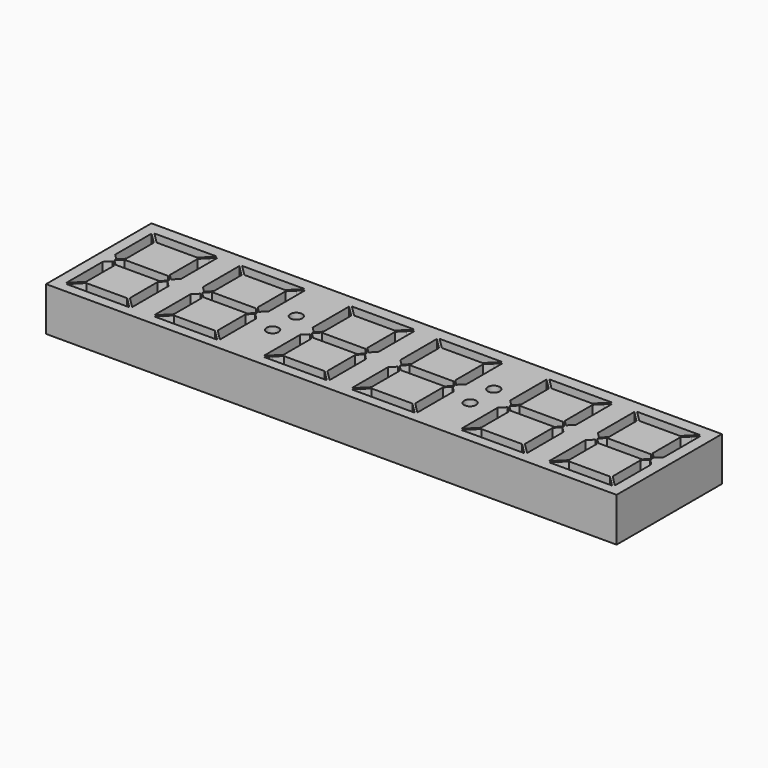
from build123d import *

# Parameters (mm, degrees)
F0_R     = 3.4648968079
F1_DEPTH = 25.4


# Not quite as in the source:
# - ends of sketch curves that miss each other by under 0.0002 mm in the source are joined


with BuildPart() as f1:
    # F0 (on Top) → F1 (new body)
    with BuildSketch(Plane.XY):
        Polygon((-45.9224169783, 52.1854245931), (-71.324658747, 52.1854245931), (-122.124658747, 52.1854245931), (-122.124658747, -24.0145754069), (-71.324658747, -24.0145754069), (-20.5201752096, -24.0145754069), (-7.824658747, -24.0145754069), (-7.8201752096, -24.0145754069), (42.975341253, -24.0145754069), (93.7798247904, -24.0145754069), (106.475341253, -24.0145754069), (106.4798247904, -24.0145754069), (157.275341253, -24.0145754069), (208.0798247904, -24.0145754069), (208.0798247904, 52.1854245931), (182.6775830217, 52.1854245931), (157.275341253, 52.1854245931), (106.4798247904, 52.1854245931), (106.475341253, 52.1854245931), (100.1298247904, 52.1854245931), (93.7798247904, 52.1854245931), (68.3775830217, 52.1854245931), (42.975341253, 52.1854245931), (-7.8201752096, 52.1854245931), (-7.824658747, 52.1854245931), (-14.1701752096, 52.1854245931), (-20.5201752096, 52.1854245931), align=None)
        Polygon((-114.8766638426, -18.2225372752), (-112.1506766486, -15.4965500813), (-108.5266638426, -11.8725372752), (-84.9227150668, -11.8725372752), (-81.2987022607, -15.4965500813), (-78.5727150668, -18.2225372752), align=None, mode=Mode.SUBTRACT)
        Polygon((-27.7726536514, -18.2225372752), (-64.0766024272, -18.2225372752), (-61.3506152332, -15.4965500813), (-57.7266024272, -11.8725372752), (-34.1226536514, -11.8725372752), (-30.4986408454, -15.4965500813), align=None, mode=Mode.SUBTRACT)
        Polygon((5.7733361574, -11.8725372752), (29.3772849332, -11.8725372752), (33.0012977393, -15.4965500813), (35.7272849332, -18.2225372752), (-0.5766638426, -18.2225372752), (2.1493233514, -15.4965500813), align=None, mode=Mode.SUBTRACT)
        Polygon((-115.7770073018, 9.0053659809), (-115.7061190955, 9.0824627244), (-112.5653735672, 12.2574627244), (-109.4246280391, 9.0824627243), (-109.4246280391, -10.9745116633), (-113.0486408451, -14.5985244694), (-115.7746284012, -17.3245116571), align=None, mode=Mode.SUBTRACT)
        Polygon((-80.8810682654, 12.2546509709), (-77.7403227372, 9.0796509709), (-77.6718137934, 9.0101770152), (-77.6718137934, -17.3273234166), (-80.3978009873, -14.6013362227), (-84.0218137919, -10.977323417), (-84.0218137936, 9.0796509708), align=None, mode=Mode.SUBTRACT)
        Polygon((-58.6275037021, -10.977323417), (-62.2515165067, -14.6013362227), (-64.9775037006, -17.3273234166), (-64.9775037006, 9.0101770152), (-64.9089947568, 9.0796509709), (-61.7682492285, 12.2546509709), (-58.6275037004, 9.0796509708), align=None, mode=Mode.SUBTRACT)
        Polygon((-112.5824693266, 13.5446828527), (-109.4275024956, 16.6996496838), (-84.0275012359, 16.699648424), (-80.866894333, 13.5446981166), (-84.0218137936, 10.349650971), (-109.4218137935, 10.349650971), (-109.4246894548, 10.3524627245), align=None, mode=Mode.SUBTRACT)
        Polygon((-61.782423161, 13.5446981166), (-58.6218162581, 16.699648424), (-33.2218162581, 16.699648424), (-30.0668481674, 13.5446828527), (-33.2246280392, 10.3524627245), (-33.2275037004, 10.349650971), (-58.6275037003, 10.349650971), align=None, mode=Mode.SUBTRACT)
        Polygon((-26.8746890928, -17.3245116571), (-29.6006766488, -14.5985244694), (-33.2246894549, -10.9745116633), (-33.2246894549, 9.0824627243), (-30.0839439267, 12.2574627244), (-26.9431983985, 9.0824627244), (-26.8723101921, 9.0053659809), align=None, mode=Mode.SUBTRACT)
        Polygon((1.7346264327, 12.2574627244), (4.8753719609, 9.0824627243), (4.8753719609, -10.9745116633), (1.2513591549, -14.5985244694), (-1.4746284012, -17.3245116571), (-1.4770073018, 9.0053659809), (-1.4061190955, 9.0824627244), align=None, mode=Mode.SUBTRACT)
        Polygon((30.2781862081, -10.977323417), (30.2781862064, 9.0796509708), (33.4189317346, 12.2546509709), (36.5596772628, 9.0796509709), (36.6281862066, 9.0101770152), (36.6281862066, -17.3273234166), (33.9021990127, -14.6013362227), align=None, mode=Mode.SUBTRACT)
        with Locations((-14.1746894548, 4.9483692275)):
            Circle(F0_R, mode=Mode.SUBTRACT)
        Polygon((1.6986249251, 13.524648424), (1.6963722036, 13.524648424), (1.6974989639, 13.5257747847), align=None, mode=Mode.SUBTRACT)
        Polygon((4.8724987641, 16.699648424), (30.2724987641, 16.699648424), (33.4160560732, 13.5617171963), (33.433105667, 13.5446981166), (33.4503257953, 13.5621060558), (33.4503719609, 13.5274627244), (33.4160560732, 13.5274627245), (30.2781862064, 10.349650971), (4.8781862065, 10.3496509707), (4.8753105452, 10.3524627245), (1.7175306734, 13.5446828527), align=None, mode=Mode.SUBTRACT)
        Polygon((52.9493847668, -15.4965500813), (56.5733975728, -11.8725372752), (80.1773463486, -11.8725372752), (83.8013591546, -15.4965500813), (86.5273463486, -18.2225372752), (50.2233975728, -18.2225372752), align=None, mode=Mode.SUBTRACT)
        Polygon((120.0733361574, -11.8725372752), (143.6772849332, -11.8725372752), (147.3012977393, -15.4965500813), (150.0272849332, -18.2225372752), (113.7233361574, -18.2225372752), (116.4493233514, -15.4965500813), align=None, mode=Mode.SUBTRACT)
        Polygon((167.2493847668, -15.4965500813), (170.8733975728, -11.8725372752), (194.4773463486, -11.8725372752), (198.1013591546, -15.4965500813), (200.8273463486, -18.2225372752), (164.5233975728, -18.2225372752), align=None, mode=Mode.SUBTRACT)
        Polygon((52.5317507714, 12.2546509709), (55.6724962996, 9.0796509708), (55.6724962979, -10.977323417), (52.0484834933, -14.6013362227), (49.3224962994, -17.3273234166), (49.3224962994, 9.0101770152), (49.3910052432, 9.0796509709), align=None, mode=Mode.SUBTRACT)
        Polygon((81.0753105451, -10.9745116633), (81.0753105451, 9.0824627243), (84.2160560733, 12.2574627244), (87.3568016015, 9.0824627244), (87.4276898079, 9.0053659809), (87.4253109084, -17.3245116571), (84.6993233512, -14.5985244694), align=None, mode=Mode.SUBTRACT)
        Polygon((116.0346264327, 12.2574627244), (119.1753719609, 9.0824627243), (119.1753719609, -10.9745116633), (115.5513591549, -14.5985244694), (112.8253715988, -17.3245116571), (112.8229926982, 9.0053659809), (112.8938809045, 9.0824627244), align=None, mode=Mode.SUBTRACT)
        Polygon((81.0724962996, 10.3496509714), (55.6724962997, 10.3496509713), (52.5346109056, 13.5274473923), (52.5003105451, 13.5274627244), (52.5003567108, 13.5621060558), (52.517576839, 13.5446981166), (52.5346264328, 13.5617171963), (55.6781837419, 16.699648424), (81.0781837419, 16.699648424), (84.2331518326, 13.5446828527), (81.0753719608, 10.3524627245), align=None, mode=Mode.SUBTRACT)
        with Locations((100.1253105452, 4.9483692275)):
            Circle(F0_R, mode=Mode.SUBTRACT)
        Polygon((84.2531835421, 13.5257747847), (84.2543103024, 13.524648424), (84.252057581, 13.524648424), align=None, mode=Mode.SUBTRACT)
        Polygon((115.9986249251, 13.5246484235), (115.9963722036, 13.5246484235), (115.9974989639, 13.5257747847), align=None, mode=Mode.SUBTRACT)
        Polygon((144.5781862081, -10.977323417), (144.5781862064, 9.0796509708), (147.7189317346, 12.2546509709), (150.8596772628, 9.0796509709), (150.9281862066, 9.0101770152), (150.9281862066, -17.3273234166), (148.2021990127, -14.6013362227), align=None, mode=Mode.SUBTRACT)
        Polygon((166.8317507714, 12.2546509709), (169.9724962996, 9.0796509708), (169.9724962979, -10.977323417), (166.3484834933, -14.6013362227), (163.6224962994, -17.3273234166), (163.6224962994, 9.0101770152), (163.6910052432, 9.0796509709), align=None, mode=Mode.SUBTRACT)
        Polygon((195.3753105451, -10.9745116633), (195.3753105451, 9.0824627243), (198.5160560733, 12.2574627244), (201.6568016015, 9.0824627244), (201.7276898079, 9.0053659809), (201.7253109084, -17.3245116571), (198.9993233512, -14.5985244694), align=None, mode=Mode.SUBTRACT)
        Polygon((119.1724987641, 16.699648424), (144.5724987641, 16.699648424), (147.7160560732, 13.5617171963), (147.733105667, 13.5446981166), (147.7503257953, 13.5621060558), (147.7503719609, 13.5274627244), (147.7160560732, 13.5274627245), (144.5781862064, 10.349650971), (119.1781862065, 10.3496509704), (119.1753105452, 10.3524627245), (116.0175306734, 13.5446828527), align=None, mode=Mode.SUBTRACT)
        Polygon((195.3724962996, 10.3496509717), (169.9724962997, 10.3496509716), (166.8346109056, 13.5274473923), (166.8003105451, 13.5274627244), (166.8003567108, 13.5621060558), (166.817576839, 13.5446981166), (166.8346264328, 13.5617171963), (169.9781837419, 16.699648424), (195.3781837419, 16.699648424), (198.5331518326, 13.5446828527), (195.3753719608, 10.3524627245), align=None, mode=Mode.SUBTRACT)
        Polygon((198.5531835421, 13.5257747847), (198.5543103024, 13.524648424), (198.552057581, 13.5246484246), align=None, mode=Mode.SUBTRACT)
        Polygon((-112.5653735672, 14.7974627245), (-115.7061190955, 17.9724627245), (-115.7748322287, 18.0419252759), (-115.7748322287, 44.3792362755), (-113.0486408451, 41.6534499185), (-109.4246280391, 38.0294371125), (-109.4246280391, 17.9724627246), align=None, mode=Mode.SUBTRACT)
        Polygon((-77.671816009, 18.0388435052), (-77.7403866174, 17.9696484239), (-80.8839439267, 14.7974627245), (-84.0275012359, 17.969648424), (-84.0275012359, 38.0266228119), (-80.3978032029, 41.650574564), (-77.671816009, 44.376561758), align=None, mode=Mode.SUBTRACT)
        Polygon((-64.977501485, 18.0388435052), (-64.977501485, 44.376561758), (-62.251514291, 41.650574564), (-58.6218162581, 38.0266228119), (-58.6218162581, 17.969648424), (-61.7653735672, 14.7974627245), (-64.9089308765, 17.9696484239), align=None, mode=Mode.SUBTRACT)
        with Locations((-14.1746894549, 22.1065562218)):
            Circle(F0_R, mode=Mode.SUBTRACT)
        Polygon((-29.6006766488, 41.6534499185), (-26.8744852653, 44.3792362755), (-26.8744852653, 18.0419252759), (-26.9431983984, 17.9724627245), (-30.0839439267, 14.7974627245), (-33.2246894549, 17.9724627246), (-33.2246894549, 38.0294371125), align=None, mode=Mode.SUBTRACT)
        Polygon((-1.4748322287, 18.0419252759), (-1.4748322287, 44.3792359067), (1.2513591549, 41.6534499185), (4.8753719609, 38.0294371125), (4.8753719609, 17.9724627246), (1.7346264328, 14.7974627245), (-1.4061190955, 17.9724627245), align=None, mode=Mode.SUBTRACT)
        Polygon((30.2724987641, 17.969648424), (30.2724987641, 38.0266228119), (33.9021967971, 41.650574564), (36.628183991, 44.376561758), (36.628183991, 18.0388435052), (36.5596133826, 17.9696484239), (33.4160560733, 14.7974627245), align=None, mode=Mode.SUBTRACT)
        Polygon((-78.572653651, 45.2774627244), (-81.298640845, 42.5514755305), (-84.9226536512, 38.9274627246), (-108.526602427, 38.9274627246), (-112.150615233, 42.5514755306), (-114.8766024268, 45.2774627244), align=None, mode=Mode.SUBTRACT)
        Polygon((-61.350676649, 42.5514755305), (-64.0766638429, 45.2774627244), (-27.7727150671, 45.2774627244), (-30.4987022609, 42.5514755306), (-34.122715067, 38.9274627246), (-57.7266638428, 38.9274627246), align=None, mode=Mode.SUBTRACT)
        Polygon((-0.5766024268, 45.2774627244), (35.727346349, 45.2774627244), (33.001359155, 42.5514755305), (29.3773463488, 38.9274627246), (5.773397573, 38.9274627246), (2.149384767, 42.5514755306), align=None, mode=Mode.SUBTRACT)
        with Locations((100.1253105451, 22.1065562218)):
            Circle(F0_R, mode=Mode.SUBTRACT)
        Polygon((49.322498515, 18.0388435052), (49.322498515, 44.376561758), (52.048485709, 41.650574564), (55.6781837419, 38.0266228119), (55.6781837419, 17.969648424), (52.5346264328, 14.7974627245), (49.3910691235, 17.9696484239), align=None, mode=Mode.SUBTRACT)
        Polygon((84.6993233512, 41.6534499185), (87.4255147347, 44.3792362755), (87.4255147347, 18.0419252759), (87.3568016016, 17.9724627245), (84.2160560733, 14.7974627245), (81.0753105451, 17.9724627246), (81.0753105451, 38.0294371125), align=None, mode=Mode.SUBTRACT)
        Polygon((112.8251677713, 18.0419252759), (112.8251677713, 44.3792359067), (115.5513591549, 41.6534499185), (119.1753719609, 38.0294371125), (119.1753719609, 17.9724627246), (116.0346264328, 14.7974627245), (112.8938809045, 17.9724627245), align=None, mode=Mode.SUBTRACT)
        Polygon((144.5724987641, 17.969648424), (144.5724987641, 38.0266228119), (148.2021967971, 41.650574564), (150.928183991, 44.376561758), (150.928183991, 18.0388435052), (150.8596133826, 17.9696484239), (147.7160560733, 14.7974627245), align=None, mode=Mode.SUBTRACT)
        Polygon((163.622498515, 18.0388435052), (163.622498515, 44.376561758), (166.348485709, 41.650574564), (169.9781837419, 38.0266228119), (169.9781837419, 17.969648424), (166.8346264328, 14.7974627245), (163.6910691235, 17.9696484239), align=None, mode=Mode.SUBTRACT)
        Polygon((198.9993233512, 41.6534499185), (201.7255147347, 44.3792362755), (201.7255147347, 18.0419252759), (201.6568016016, 17.9724627245), (198.5160560733, 14.7974627245), (195.3753105451, 17.9724627246), (195.3753105451, 38.0294371125), align=None, mode=Mode.SUBTRACT)
        Polygon((80.177284933, 38.9274627246), (56.5733361572, 38.9274627246), (52.949323351, 42.5514755305), (50.2233361571, 45.2774627244), (86.5272849329, 45.2774627244), (83.8012977391, 42.5514755306), align=None, mode=Mode.SUBTRACT)
        Polygon((113.7233975732, 45.2774627244), (150.027346349, 45.2774627244), (147.301359155, 42.5514755305), (143.6773463488, 38.9274627246), (120.073397573, 38.9274627246), (116.449384767, 42.5514755306), align=None, mode=Mode.SUBTRACT)
        Polygon((194.477284933, 38.9274627246), (170.8733361572, 38.9274627246), (167.249323351, 42.5514755305), (164.5233361571, 45.2774627244), (200.8272849329, 45.2774627244), (198.1012977391, 42.5514755306), align=None, mode=Mode.SUBTRACT)
    extrude(amount=F1_DEPTH)


solid = f1.part
